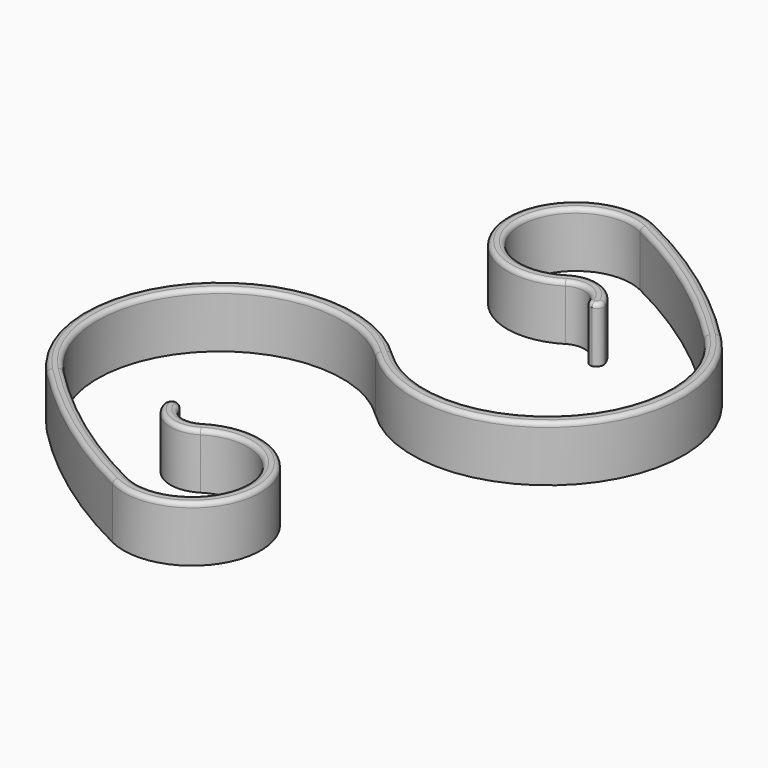
from build123d import *

# Parameters (mm, degrees)
F1_DEPTH     = 7.5
F2_T1_DEPTH  = 27.7443791337
F2_T3_DEPTH  = 23.7298334621
F3_T3_ANGLE  = 178.6060541067
F3_T6_ANGLE  = 178.6060541067
F3_T9_ANGLE  = 178.6060541067
F3_T12_ANGLE = 19.3744330298
F3_T15_ANGLE = 238.2179683188
F3_T18_ANGLE = 102.3234179936
F3_T21_ANGLE = 155.5482640924
F3_T24_ANGLE = 19.3744330298
F3_T27_ANGLE = 238.2179683188
F3_T30_ANGLE = 101.5434068893
F3_T33_ANGLE = 185.3047109678
F3_T36_ANGLE = 19.3744330298
F3_T39_ANGLE = 178.6060541067
F3_T42_ANGLE = 19.3744330298
F3_T45_ANGLE = 238.2179683188
F3_T48_ANGLE = 102.3234179936
F3_T51_ANGLE = 155.5482640924
F3_T54_ANGLE = 238.2179683188
F3_T57_ANGLE = 101.5434068893
F3_T60_ANGLE = 185.3047109678


# Not quite as in the source:
# - a fillet or chamfer that OpenCascade refuses, or shapes differently, is made with other operations: its cross-section is extruded or revolved along the edge and cut away or added


with BuildPart() as f1:
    # F0 (on Top) → F1 (new body, symmetric)
    with BuildSketch(Plane.XY):
        with BuildLine():
            ThreePointArc((7.925558911, 52.2647922691), (-14.9822650032, 64.2707981257), (6.6513574574, 78.4446808803))
            ThreePointArc((6.6513574574, 78.4446808803), (28.7100701018, 65.1032562904), (48.2092941819, 48.2402591103))
            ThreePointArc((48.2092941819, 48.2402591103), (47.925443489, 1.572031194), (1.2572155727, 1.2881805012))
            ThreePointArc((1.2572155727, 1.2881805012), (-50.4710279013, 0.9735532183), (-50.7856551842, -50.7546902558))
            ThreePointArc((-50.7856551842, -50.7546902558), (-30.8265929187, -68.0153571069), (-8.2476832472, -81.6714042916))
            ThreePointArc((-8.2476832472, -81.6714042916), (18.578008604, -64.0957896758), (-9.8276930496, -49.2083424137))
            ThreePointArc((-9.8276930496, -49.2083424137), (-15.6755755072, -49.4836301273), (-18.9742141949, -44.6470512362))
            Line((-18.9742141949, -44.6470512362), (-22.5599927435, -44.9667263851))
            ThreePointArc((-22.5599927435, -44.9667263851), (-17.2821708431, -52.7052526109), (-7.925558911, -52.2647922691))
            ThreePointArc((-7.925558911, -52.2647922691), (14.9822650032, -64.2707981257), (-6.6513574574, -78.4446808803))
            ThreePointArc((-6.6513574574, -78.4446808803), (-28.7100701018, -65.1032562904), (-48.2092941819, -48.2402591103))
            ThreePointArc((-48.2092941819, -48.2402591103), (-47.925443489, -1.572031194), (-1.2572155727, -1.2881805012))
            ThreePointArc((-1.2572155727, -1.2881805012), (50.4710279013, -0.9735532183), (50.7856551842, 50.7546902558))
            ThreePointArc((50.7856551842, 50.7546902558), (30.8265929187, 68.0153571069), (8.2476832472, 81.6714042916))
            ThreePointArc((8.2476832472, 81.6714042916), (-18.578008604, 64.0957896758), (9.8276930496, 49.2083424137))
            ThreePointArc((9.8276930496, 49.2083424137), (15.6755755072, 49.4836301273), (18.9742141949, 44.6470512362))
            Line((18.9742141949, 44.6470512362), (22.5599927435, 44.9667263851))
            ThreePointArc((22.5599927435, 44.9667263851), (17.2821708431, 52.7052526109), (7.925558911, 52.2647922691))
        make_face()
    extrude(amount=F1_DEPTH, both=True)

    # F2: fillet of radius 2 on 4 edges, made by hand

    # F2_s2 → F2_t1 (cut)
    with BuildSketch(Plane.XY.offset(-13.8721895669)):
        with BuildLine():
            ThreePointArc((21.9986226844, 47.4530151127), (21.8144329663, 45.6894226659), (20.3010728914, 44.7653417959))
            Line((20.3010728914, 44.7653417959), (22.5599927435, 44.9667263851))
            ThreePointArc((22.5599927435, 44.9667263851), (22.3621906734, 46.2285845899), (21.9986226844, 47.4530151127))
        make_face()
        with BuildLine():
            ThreePointArc((-21.9986226844, -47.4530151127), (-21.8144329663, -45.6894226659), (-20.3010728914, -44.7653417959))
            Line((-20.3010728914, -44.7653417959), (-22.5599927435, -44.9667263851))
            ThreePointArc((-22.5599927435, -44.9667263851), (-22.3621906734, -46.2285845899), (-21.9986226844, -47.4530151127))
        make_face()
    extrude(amount=F2_T1_DEPTH, mode=Mode.SUBTRACT)

    # F2_s4 → F2_t3 (cut)
    with BuildSketch(Plane.XY.offset(-11.864916731)):
        with BuildLine():
            ThreePointArc((20.713283615, 44.8020907258), (19.4561826722, 45.110541531), (18.651243886, 46.1242072699))
            ThreePointArc((18.651243886, 46.1242072699), (18.8594472197, 45.3958438712), (18.9742141949, 44.6470512362))
            Line((18.9742141949, 44.6470512362), (20.713283615, 44.8020907258))
        make_face()
        with BuildLine():
            ThreePointArc((-20.713283615, -44.8020907258), (-19.4561826722, -45.110541531), (-18.651243886, -46.1242072699))
            ThreePointArc((-18.651243886, -46.1242072699), (-18.8594472197, -45.3958438712), (-18.9742141949, -44.6470512362))
            Line((-18.9742141949, -44.6470512362), (-20.713283615, -44.8020907258))
        make_face()
    extrude(amount=F2_T3_DEPTH, mode=Mode.SUBTRACT)

    # F3: fillet of radius 1.2 on 2 edges, made by hand


with BuildPart() as f3_tool1:
    # F3_s2 → F3_t3 (revolve)
    with BuildSketch(Plane(origin=(0.5947272864, -0.6093752818, 0), x_dir=(0, 0, 1), z_dir=(0.698453096, -0.715655834, 0))):
        with BuildLine():
            ThreePointArc((7.5, 69.39482096), (7.1485281374, 68.5462928226), (6.3, 68.19482096))
            Line((6.3, 68.19482096), (7.5, 68.19482096))
            Line((7.5, 68.19482096), (7.5, 69.39482096))
        make_face()
    revolve(axis=Axis((-24.447667151, -25.0498075321, 7.5), (0, 0, -1)), revolution_arc=F3_T3_ANGLE)


with BuildPart() as f3_tool4:
    # F3_s5 → F3_t6 (revolve)
    with BuildSketch(Plane(origin=(0, 0, 0), x_dir=(0, 0, 1), z_dir=(0.715655834, -0.698453096, 0))):
        with BuildLine():
            ThreePointArc((7.5, -0.6), (7.1485281374, -1.4485281374), (6.3, -1.8))
            Line((6.3, -1.8), (7.5, -1.8))
            Line((7.5, -1.8), (7.5, -0.6))
        make_face()
    revolve(axis=Axis((-24.447667151, -25.0498075321, 7.5), (0, 0, 1)), revolution_arc=F3_T6_ANGLE)


with BuildPart() as f3_tool7:
    # F3_s8 → F3_t9 (revolve)
    with BuildSketch(Plane(origin=(-0.5947272864, 0.6093752818, 0), x_dir=(0, 0, 1), z_dir=(-0.698453096, 0.715655834, 0))):
        with BuildLine():
            ThreePointArc((7.5, 69.39482096), (7.1485281374, 68.5462928226), (6.3, 68.19482096))
            Line((6.3, 68.19482096), (7.5, 68.19482096))
            Line((7.5, 68.19482096), (7.5, 69.39482096))
        make_face()
    revolve(axis=Axis((24.447667151, 25.0498075321, 7.5), (0, 0, -1)), revolution_arc=F3_T9_ANGLE)


with BuildPart() as f3_tool10:
    # F3_s11 → F3_t12 (revolve)
    with BuildSketch(Plane(origin=(0.5947272864, -0.6093752818, 0), x_dir=(0, 0, 1), z_dir=(-0.698453096, 0.715655834, 0))):
        with BuildLine():
            ThreePointArc((7.5, -70.59482096), (7.1485281374, -71.4433490974), (6.3, -71.79482096))
            Line((6.3, -71.79482096), (7.5, -71.79482096))
            Line((7.5, -71.79482096), (7.5, -70.59482096))
        make_face()
    revolve(axis=Axis((61.0400941451, 58.3830224798, 7.5), (0, 0, 1)), revolution_arc=F3_T12_ANGLE)


with BuildPart() as f3_tool13:
    # F3_s14 → F3_t15 (revolve)
    with BuildSketch(Plane(origin=(25.8339982147, -12.7806050742, 0), x_dir=(0, 0, 1), z_dir=(-0.8963120587, 0.4434238305, 0))):
        with BuildLine():
            ThreePointArc((7.5, -75.6602838148), (7.1485281374, -76.5088119522), (6.3, -76.8602838148))
            Line((6.3, -76.8602838148), (7.5, -76.8602838148))
            Line((7.5, -76.8602838148), (7.5, -75.6602838148))
        make_face()
    revolve(axis=Axis((0, -65, 7.5), (0, 0, 1)), revolution_arc=F3_T15_ANGLE)


with BuildPart() as f3_tool16:
    # F3_s17 → F3_t18 (revolve)
    with BuildSketch(Plane(origin=(-29.1586068554, -18.1464065038, 0), x_dir=(0, 0, 1), z_dir=(0.8490138487, 0.5283705941, 0))):
        with BuildLine():
            ThreePointArc((7.5, 37.7859001671), (7.1485281374, 36.9373720297), (6.3, 36.5859001671))
            Line((6.3, 36.5859001671), (7.5, 36.5859001671))
            Line((7.5, 36.5859001671), (7.5, 37.7859001671))
        make_face()
    revolve(axis=Axis((-12.997916614, -44.1142593214, 7.5), (0, 0, -1)), revolution_arc=F3_T18_ANGLE)


with BuildPart() as f3_tool19:
    # F3_s20 → F3_t21 (revolve)
    with BuildSketch(Plane(origin=(-4.1146850802, -48.1961131121, 0), x_dir=(0, 0, 1), z_dir=(-0.0850643542, -0.9963754592, 0))):
        with BuildLine():
            ThreePointArc((7.5, 17.2807363317), (7.1485281374, 18.1292644691), (6.3, 18.4807363317))
            Line((6.3, 18.4807363317), (7.5, 18.4807363317))
            Line((7.5, 18.4807363317), (7.5, 17.2807363317))
        make_face()
    revolve(axis=Axis((-20.5356863101, -46.7941899196, 7.5), (0, 0, -1)), revolution_arc=F3_T21_ANGLE)


with BuildPart() as f3_tool22:
    # F3_s23 → F3_t24 (revolve)
    with BuildSketch(Plane(origin=(-25.8339982147, 12.7806050742, 0), x_dir=(0, 0, 1), z_dir=(-0.8963120587, 0.4434238305, 0))):
        with BuildLine():
            ThreePointArc((7.5, 74.4602838148), (7.1485281374, 73.6117556774), (6.3, 73.2602838148))
            Line((6.3, 73.2602838148), (7.5, 73.2602838148))
            Line((7.5, 73.2602838148), (7.5, 74.4602838148))
        make_face()
    revolve(axis=Axis((-61.0400941451, -58.3830224798, 7.5), (0, 0, -1)), revolution_arc=F3_T24_ANGLE)


with BuildPart() as f3_tool25:
    # F3_s26 → F3_t27 (revolve)
    with BuildSketch(Plane(origin=(29.1586068554, 18.1464065038, 0), x_dir=(0, 0, 1), z_dir=(0.8490138487, 0.5283705941, 0))):
        with BuildLine():
            ThreePointArc((7.5, -38.9859001671), (7.1485281374, -39.8344283045), (6.3, -40.1859001671))
            Line((6.3, -40.1859001671), (7.5, -40.1859001671))
            Line((7.5, -40.1859001671), (7.5, -38.9859001671))
        make_face()
    revolve(axis=Axis((0, 65, 7.5), (0, 0, -1)), revolution_arc=F3_T27_ANGLE)


with BuildPart() as f3_tool28:
    # F3_s29 → F3_t30 (revolve)
    with BuildSketch(Plane(origin=(-12.8124250757, 34.5400740165, 0), x_dir=(0, 0, 1), z_dir=(0.3477870616, -0.937573549, 0))):
        with BuildLine():
            ThreePointArc((7.5, -35.9288714334), (7.1485281374, -36.7773995708), (6.3, -37.1288714334))
            Line((6.3, -37.1288714334), (7.5, -37.1288714334))
            Line((7.5, -37.1288714334), (7.5, -35.9288714334))
        make_face()
    revolve(axis=Axis((12.997916614, 44.1142593214, 7.5), (0, 0, 1)), revolution_arc=F3_T30_ANGLE)


with BuildPart() as f3_tool31:
    # F3_s32 → F3_t33 (revolve)
    with BuildSketch(Plane(origin=(-12.812425077, 34.5400740137, 0), x_dir=(0, 0, 1), z_dir=(-0.3477870617, 0.937573549, 0))):
        with BuildLine():
            ThreePointArc((7.5, 35.9288714354), (7.1485281374, 36.7773995729), (6.3, 37.1288714354))
            Line((6.3, 37.1288714354), (7.5, 37.1288714354))
            Line((7.5, 37.1288714354), (7.5, 35.9288714354))
        make_face()
    revolve(axis=Axis((20.1234755865, 46.7574409894, 7.5), (0, 0, -1)), revolution_arc=F3_T33_ANGLE)


with BuildPart() as f3_tool34:
    # F3_s35 → F3_t36 (revolve)
    with BuildSketch(Plane(origin=(25.8339982147, -12.7806050742, 0), x_dir=(0, 0, 1), z_dir=(0.8963120587, -0.4434238305, 0))):
        with BuildLine():
            ThreePointArc((7.5, 74.4602838148), (7.1485281374, 73.6117556774), (6.3, 73.2602838148))
            Line((6.3, 73.2602838148), (7.5, 73.2602838148))
            Line((7.5, 73.2602838148), (7.5, 74.4602838148))
        make_face()
    revolve(axis=Axis((61.0400941451, 58.3830224798, 7.5), (0, 0, -1)), revolution_arc=F3_T36_ANGLE)


with BuildPart() as f3_tool37:
    # F3_s38 → F3_t39 (revolve)
    with BuildSketch(Plane(origin=(0, 0, 0), x_dir=(0, 0, 1), z_dir=(-0.715655834, 0.698453096, 0))):
        with BuildLine():
            ThreePointArc((7.5, -0.6), (7.1485281374, -1.4485281374), (6.3, -1.8))
            Line((6.3, -1.8), (7.5, -1.8))
            Line((7.5, -1.8), (7.5, -0.6))
        make_face()
    revolve(axis=Axis((24.447667151, 25.0498075321, 7.5), (0, 0, 1)), revolution_arc=F3_T39_ANGLE)


with BuildPart() as f3_tool40:
    # F3_s41 → F3_t42 (revolve)
    with BuildSketch(Plane(origin=(-0.5947272864, 0.6093752818, 0), x_dir=(0, 0, 1), z_dir=(0.698453096, -0.715655834, 0))):
        with BuildLine():
            ThreePointArc((7.5, -70.59482096), (7.1485281374, -71.4433490974), (6.3, -71.79482096))
            Line((6.3, -71.79482096), (7.5, -71.79482096))
            Line((7.5, -71.79482096), (7.5, -70.59482096))
        make_face()
    revolve(axis=Axis((-61.0400941451, -58.3830224798, 7.5), (0, 0, 1)), revolution_arc=F3_T42_ANGLE)


with BuildPart() as f3_tool43:
    # F3_s44 → F3_t45 (revolve)
    with BuildSketch(Plane(origin=(-25.8339982147, 12.7806050742, 0), x_dir=(0, 0, 1), z_dir=(0.8963120587, -0.4434238305, 0))):
        with BuildLine():
            ThreePointArc((6.3, -76.8602838148), (7.1485281374, -76.5088119522), (7.5, -75.6602838148))
            Line((7.5, -75.6602838148), (7.5, -76.8602838148))
            Line((7.5, -76.8602838148), (6.3, -76.8602838148))
        make_face()
    revolve(axis=Axis((0, 65, 7.5), (0, 0, 1)), revolution_arc=F3_T45_ANGLE)


with BuildPart() as f3_tool46:
    # F3_s47 → F3_t48 (revolve)
    with BuildSketch(Plane(origin=(29.1586068554, 18.1464065038, 0), x_dir=(0, 0, 1), z_dir=(-0.8490138487, -0.5283705941, 0))):
        with BuildLine():
            ThreePointArc((6.3, 36.5859001671), (7.1485281374, 36.9373720297), (7.5, 37.7859001671))
            Line((7.5, 37.7859001671), (7.5, 36.5859001671))
            Line((7.5, 36.5859001671), (6.3, 36.5859001671))
        make_face()
    revolve(axis=Axis((12.997916614, 44.1142593214, 7.5), (0, 0, -1)), revolution_arc=F3_T48_ANGLE)


with BuildPart() as f3_tool49:
    # F3_s50 → F3_t51 (revolve)
    with BuildSketch(Plane(origin=(4.1146850802, 48.1961131121, 0), x_dir=(0, 0, 1), z_dir=(0.0850643542, 0.9963754592, 0))):
        with BuildLine():
            ThreePointArc((7.5, 17.2807363317), (7.1485281374, 18.1292644691), (6.3, 18.4807363317))
            Line((6.3, 18.4807363317), (7.5, 18.4807363317))
            Line((7.5, 18.4807363317), (7.5, 17.2807363317))
        make_face()
    revolve(axis=Axis((20.5356863101, 46.7941899196, 7.5), (0, 0, -1)), revolution_arc=F3_T51_ANGLE)


with BuildPart() as f3_tool52:
    # F3_s53 → F3_t54 (revolve)
    with BuildSketch(Plane(origin=(-29.1586068554, -18.1464065038, 0), x_dir=(0, 0, 1), z_dir=(-0.8490138487, -0.5283705941, 0))):
        with BuildLine():
            ThreePointArc((7.5, -38.9859001671), (7.1485281374, -39.8344283045), (6.3, -40.1859001671))
            Line((6.3, -40.1859001671), (7.5, -40.1859001671))
            Line((7.5, -40.1859001671), (7.5, -38.9859001671))
        make_face()
    revolve(axis=Axis((0, -65, 7.5), (0, 0, -1)), revolution_arc=F3_T54_ANGLE)


with BuildPart() as f3_tool55:
    # F3_s56 → F3_t57 (revolve)
    with BuildSketch(Plane(origin=(12.8124250757, -34.5400740165, 0), x_dir=(0, 0, 1), z_dir=(-0.3477870616, 0.937573549, 0))):
        with BuildLine():
            ThreePointArc((7.5, -35.9288714334), (7.1485281374, -36.7773995708), (6.3, -37.1288714334))
            Line((6.3, -37.1288714334), (7.5, -37.1288714334))
            Line((7.5, -37.1288714334), (7.5, -35.9288714334))
        make_face()
    revolve(axis=Axis((-12.997916614, -44.1142593214, 7.5), (0, 0, 1)), revolution_arc=F3_T57_ANGLE)


with BuildPart() as f3_tool58:
    # F3_s59 → F3_t60 (revolve)
    with BuildSketch(Plane(origin=(12.812425077, -34.5400740137, 0), x_dir=(0, 0, 1), z_dir=(0.3477870617, -0.937573549, 0))):
        with BuildLine():
            ThreePointArc((7.5, 35.9288714354), (7.1485281374, 36.7773995729), (6.3, 37.1288714354))
            Line((6.3, 37.1288714354), (7.5, 37.1288714354))
            Line((7.5, 37.1288714354), (7.5, 35.9288714354))
        make_face()
    revolve(axis=Axis((-20.1234755865, -46.7574409894, 7.5), (0, 0, -1)), revolution_arc=F3_T60_ANGLE)


with BuildPart() as f1_1:
    add(f1.part)

    # F3_t61: cut F3_tool1, F3_tool4, F3_tool7, F3_tool10, F3_tool13, F3_tool16, F3_tool19, F3_tool22, F3_tool25, F3_tool28, F3_tool31, F3_tool34, F3_tool37, F3_tool40, F3_tool43, F3_tool46, F3_tool49, F3_tool52, F3_tool55, F3_tool58
    add([f3_tool1.part, f3_tool4.part, f3_tool7.part, f3_tool10.part, f3_tool13.part, f3_tool16.part, f3_tool19.part, f3_tool22.part, f3_tool25.part, f3_tool28.part, f3_tool31.part, f3_tool34.part, f3_tool37.part, f3_tool40.part, f3_tool43.part, f3_tool46.part, f3_tool49.part, f3_tool52.part, f3_tool55.part, f3_tool58.part], mode=Mode.SUBTRACT)


solid = f1_1.part
